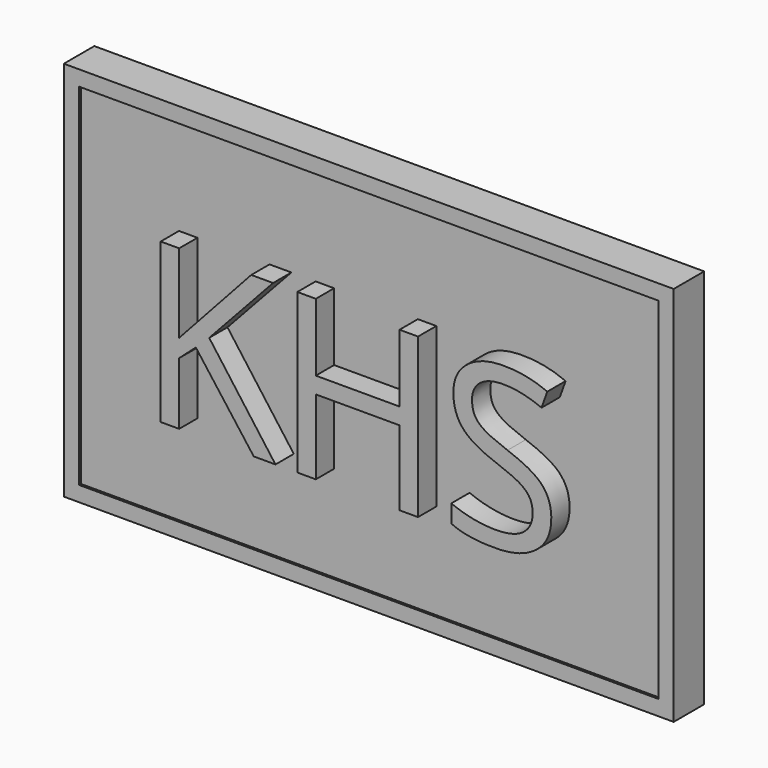
from build123d import *

# Parameters (mm, degrees)
F0_W         = 400
F0_H         = 250
F1_DEPTH     = 25
F2_W         = 380
F2_H         = 230
F3_DEPTH     = 1.5
F4_W         = 300
F4_H         = 150
F5_DEPTH     = 25
F6_R         = 15
F7_DEPTH     = 30
F8_TEXT_SIZE = 146.0353679407
F9_DEPTH     = 15


# Not quite as in the source:
# - Text() gives the source's letters only with a copy of the font that has no kerning and outlines rounded to 1/6400 em; it was checked with that copy


with BuildPart() as f1:
    # F0 (on Front) → F1 (new body)
    with BuildSketch(Plane.XZ):
        Rectangle(F0_W, F0_H)
    extrude(amount=F1_DEPTH)

    # F2 (on face) → F3 (cut)
    with BuildSketch(Plane.XZ.offset(25)):
        Rectangle(F2_W, F2_H)
    extrude(amount=-F3_DEPTH, mode=Mode.SUBTRACT)

    # F4 (on face) → F5 (join)
    with BuildSketch(Plane(origin=(0, 0, 0), x_dir=(-1, 0, 0), z_dir=(0, 1, 0))):
        Rectangle(F4_W, F4_H)
    extrude(amount=F5_DEPTH)

    # F6 (on face) → F7 (join)
    with BuildSketch(Plane(origin=(0, 25, 0), x_dir=(-1, 0, 0), z_dir=(0, 1, 0))):
        Circle(F6_R)
    extrude(amount=F7_DEPTH)

    # F8 (on face) → F9 (join)
    with BuildSketch(Plane.XZ.offset(23.5)):
        with Locations((-140, -52.2668613109)):
            Text('KHS', F8_TEXT_SIZE, font='Open Sans', text_align=(TextAlign.LEFT, TextAlign.BOTTOM))
    extrude(amount=F9_DEPTH)


solid = f1.part
